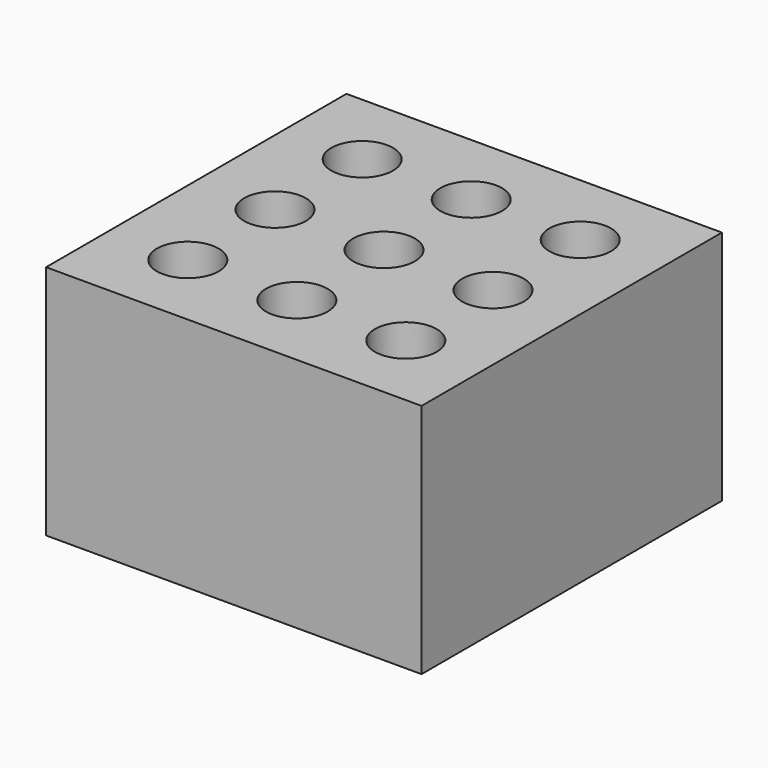
from build123d import *

# Parameters (mm, degrees)
F0_W      = 62
F0_H      = 62
F1_DEPTH  = 39
F4_DEPTH  = 8
F4_TAPER  = 22
F6_DEPTH  = 6
F6_TAPER  = 18
F9_DEPTH  = 6
F11_R     = 5.1
F12_DEPTH = 19


with BuildPart() as f1:
    # F0 (on Top) → F1 (new body)
    with BuildSketch(Plane.XY):
        Rectangle(F0_W, F0_H)
    extrude(amount=F1_DEPTH)

    # F3 (on Top) → F4 (cut)
    with BuildSketch(Plane.XY):
        with BuildLine():
            ThreePointArc((30.5, 29), (30.06066, 30.06066), (29, 30.5))
            Line((29, 30.5), (-29, 30.5))
            ThreePointArc((-29, 30.5), (-30.06066, 30.06066), (-30.5, 29))
            Line((-30.5, 29), (-30.5, -29))
            ThreePointArc((-30.5, -29), (-30.06066, -30.06066), (-29, -30.5))
            Line((-29, -30.5), (29, -30.5))
            ThreePointArc((29, -30.5), (30.06066, -30.06066), (30.5, -29))
            Line((30.5, -29), (30.5, 29))
        make_face()
    extrude(amount=F4_DEPTH, taper=F4_TAPER, mode=Mode.SUBTRACT)

    # F5 (on offset) → F6 (cut)
    with BuildSketch(Plane.XY.offset(8)):
        with BuildLine():
            Line((-9.5, -24.5), (-9.5, -11.5))
            ThreePointArc((-9.5, -11.5), (-10.085786, -10.085786), (-11.5, -9.5))
            Line((-11.5, -9.5), (-24.5, -9.5))
            ThreePointArc((-24.5, -9.5), (-25.914214, -10.085786), (-26.5, -11.5))
            Line((-26.5, -11.5), (-26.5, -24.5))
            ThreePointArc((-26.5, -24.5), (-25.914214, -25.914214), (-24.5, -26.5))
            Line((-24.5, -26.5), (-11.5, -26.5))
            ThreePointArc((-11.5, -26.5), (-10.085786, -25.914214), (-9.5, -24.5))
        make_face()
        with BuildLine():
            Line((8.5, -24.5), (8.5, -11.5))
            ThreePointArc((8.5, -11.5), (7.914214, -10.085786), (6.5, -9.5))
            Line((6.5, -9.5), (-6.5, -9.5))
            ThreePointArc((-6.5, -9.5), (-7.914214, -10.085786), (-8.5, -11.5))
            Line((-8.5, -11.5), (-8.5, -24.5))
            ThreePointArc((-8.5, -24.5), (-7.914214, -25.914214), (-6.5, -26.5))
            Line((-6.5, -26.5), (6.5, -26.5))
            ThreePointArc((6.5, -26.5), (7.914214, -25.914214), (8.5, -24.5))
        make_face()
        with BuildLine():
            Line((24.5, -9.5), (11.5, -9.5))
            ThreePointArc((11.5, -9.5), (10.085786, -10.085786), (9.5, -11.5))
            Line((9.5, -11.5), (9.5, -24.5))
            ThreePointArc((9.5, -24.5), (10.085786, -25.914214), (11.5, -26.5))
            Line((11.5, -26.5), (24.5, -26.5))
            ThreePointArc((24.5, -26.5), (25.914214, -25.914214), (26.5, -24.5))
            Line((26.5, -24.5), (26.5, -11.5))
            ThreePointArc((26.5, -11.5), (25.914214, -10.085786), (24.5, -9.5))
        make_face()
        with BuildLine():
            Line((26.5, -6.5), (26.5, 6.5))
            ThreePointArc((26.5, 6.5), (25.914214, 7.914214), (24.5, 8.5))
            Line((24.5, 8.5), (11.5, 8.5))
            ThreePointArc((11.5, 8.5), (10.085786, 7.914214), (9.5, 6.5))
            Line((9.5, 6.5), (9.5, -6.5))
            ThreePointArc((9.5, -6.5), (10.085786, -7.914214), (11.5, -8.5))
            Line((11.5, -8.5), (24.5, -8.5))
            ThreePointArc((24.5, -8.5), (25.914214, -7.914214), (26.5, -6.5))
        make_face()
        with BuildLine():
            Line((8.5, -6.5), (8.5, 6.5))
            ThreePointArc((8.5, 6.5), (7.914214, 7.914214), (6.5, 8.5))
            Line((6.5, 8.5), (-6.5, 8.5))
            ThreePointArc((-6.5, 8.5), (-7.914214, 7.914214), (-8.5, 6.5))
            Line((-8.5, 6.5), (-8.5, -6.5))
            ThreePointArc((-8.5, -6.5), (-7.914214, -7.914214), (-6.5, -8.5))
            Line((-6.5, -8.5), (6.5, -8.5))
            ThreePointArc((6.5, -8.5), (7.914214, -7.914214), (8.5, -6.5))
        make_face()
        with BuildLine():
            Line((-9.5, -6.5), (-9.5, 6.5))
            ThreePointArc((-9.5, 6.5), (-10.085786, 7.914214), (-11.5, 8.5))
            Line((-11.5, 8.5), (-24.5, 8.5))
            ThreePointArc((-24.5, 8.5), (-25.914214, 7.914214), (-26.5, 6.5))
            Line((-26.5, 6.5), (-26.5, -6.5))
            ThreePointArc((-26.5, -6.5), (-25.914214, -7.914214), (-24.5, -8.5))
            Line((-24.5, -8.5), (-11.5, -8.5))
            ThreePointArc((-11.5, -8.5), (-10.085786, -7.914214), (-9.5, -6.5))
        make_face()
        with BuildLine():
            Line((-9.5, 11.5), (-9.5, 24.5))
            ThreePointArc((-9.5, 24.5), (-10.085786, 25.914214), (-11.5, 26.5))
            Line((-11.5, 26.5), (-24.5, 26.5))
            ThreePointArc((-24.5, 26.5), (-25.914214, 25.914214), (-26.5, 24.5))
            Line((-26.5, 24.5), (-26.5, 11.5))
            ThreePointArc((-26.5, 11.5), (-25.914214, 10.085786), (-24.5, 9.5))
            Line((-24.5, 9.5), (-11.5, 9.5))
            ThreePointArc((-11.5, 9.5), (-10.085786, 10.085786), (-9.5, 11.5))
        make_face()
        with BuildLine():
            Line((8.5, 11.5), (8.5, 24.5))
            ThreePointArc((8.5, 24.5), (7.914214, 25.914214), (6.5, 26.5))
            Line((6.5, 26.5), (-6.5, 26.5))
            ThreePointArc((-6.5, 26.5), (-7.914214, 25.914214), (-8.5, 24.5))
            Line((-8.5, 24.5), (-8.5, 11.5))
            ThreePointArc((-8.5, 11.5), (-7.914214, 10.085786), (-6.5, 9.5))
            Line((-6.5, 9.5), (6.5, 9.5))
            ThreePointArc((6.5, 9.5), (7.914214, 10.085786), (8.5, 11.5))
        make_face()
        with BuildLine():
            Line((26.5, 11.5), (26.5, 24.5))
            ThreePointArc((26.5, 24.5), (25.914214, 25.914214), (24.5, 26.5))
            Line((24.5, 26.5), (11.5, 26.5))
            ThreePointArc((11.5, 26.5), (10.085786, 25.914214), (9.5, 24.5))
            Line((9.5, 24.5), (9.5, 11.5))
            ThreePointArc((9.5, 11.5), (10.085786, 10.085786), (11.5, 9.5))
            Line((11.5, 9.5), (24.5, 9.5))
            ThreePointArc((24.5, 9.5), (25.914214, 10.085786), (26.5, 11.5))
        make_face()
    extrude(amount=F6_DEPTH, taper=F6_TAPER, mode=Mode.SUBTRACT)

    # F8 (on offset) → F9 (cut)
    with BuildSketch(Plane.XY.offset(14)):
        with BuildLine():
            ThreePointArc((11.55, -23.45), (11.842893, -24.157107), (12.55, -24.45))
            Line((12.55, -24.45), (23.45, -24.45))
            ThreePointArc((23.45, -24.45), (24.157107, -24.157107), (24.45, -23.45))
            Line((24.45, -23.45), (24.45, -12.55))
            ThreePointArc((24.45, -12.55), (24.157107, -11.842893), (23.45, -11.55))
            Line((23.45, -11.55), (12.55, -11.55))
            ThreePointArc((12.55, -11.55), (11.842893, -11.842893), (11.55, -12.55))
            Line((11.55, -12.55), (11.55, -23.45))
        make_face()
        with BuildLine():
            Line((11.55, 5.45), (11.55, -5.45))
            ThreePointArc((11.55, -5.45), (11.842893, -6.157107), (12.55, -6.45))
            Line((12.55, -6.45), (23.45, -6.45))
            ThreePointArc((23.45, -6.45), (24.157107, -6.157107), (24.45, -5.45))
            Line((24.45, -5.45), (24.45, 5.45))
            ThreePointArc((24.45, 5.45), (24.157107, 6.157107), (23.45, 6.45))
            Line((23.45, 6.45), (12.55, 6.45))
            ThreePointArc((12.55, 6.45), (11.842893, 6.157107), (11.55, 5.45))
        make_face()
        with BuildLine():
            Line((11.55, 23.45), (11.55, 12.55))
            ThreePointArc((11.55, 12.55), (11.842893, 11.842893), (12.55, 11.55))
            Line((12.55, 11.55), (23.45, 11.55))
            ThreePointArc((23.45, 11.55), (24.157107, 11.842893), (24.45, 12.55))
            Line((24.45, 12.55), (24.45, 23.45))
            ThreePointArc((24.45, 23.45), (24.157107, 24.157107), (23.45, 24.45))
            Line((23.45, 24.45), (12.55, 24.45))
            ThreePointArc((12.55, 24.45), (11.842893, 24.157107), (11.55, 23.45))
        make_face()
        with BuildLine():
            Line((-6.45, -12.55), (-6.45, -23.45))
            ThreePointArc((-6.45, -23.45), (-6.157107, -24.157107), (-5.45, -24.45))
            Line((-5.45, -24.45), (5.45, -24.45))
            ThreePointArc((5.45, -24.45), (6.157107, -24.157107), (6.45, -23.45))
            Line((6.45, -23.45), (6.45, -12.55))
            ThreePointArc((6.45, -12.55), (6.157107, -11.842893), (5.45, -11.55))
            Line((5.45, -11.55), (-5.45, -11.55))
            ThreePointArc((-5.45, -11.55), (-6.157107, -11.842893), (-6.45, -12.55))
        make_face()
        with BuildLine():
            Line((-6.45, 5.45), (-6.45, -5.45))
            ThreePointArc((-6.45, -5.45), (-6.157107, -6.157107), (-5.45, -6.45))
            Line((-5.45, -6.45), (5.45, -6.45))
            ThreePointArc((5.45, -6.45), (6.157107, -6.157107), (6.45, -5.45))
            Line((6.45, -5.45), (6.45, 5.45))
            ThreePointArc((6.45, 5.45), (6.157107, 6.157107), (5.45, 6.45))
            Line((5.45, 6.45), (-5.45, 6.45))
            ThreePointArc((-5.45, 6.45), (-6.157107, 6.157107), (-6.45, 5.45))
        make_face()
        with BuildLine():
            Line((-6.45, 23.45), (-6.45, 12.55))
            ThreePointArc((-6.45, 12.55), (-6.157107, 11.842893), (-5.45, 11.55))
            Line((-5.45, 11.55), (5.45, 11.55))
            ThreePointArc((5.45, 11.55), (6.157107, 11.842893), (6.45, 12.55))
            Line((6.45, 12.55), (6.45, 23.45))
            ThreePointArc((6.45, 23.45), (6.157107, 24.157107), (5.45, 24.45))
            Line((5.45, 24.45), (-5.45, 24.45))
            ThreePointArc((-5.45, 24.45), (-6.157107, 24.157107), (-6.45, 23.45))
        make_face()
        with BuildLine():
            Line((-24.45, -12.55), (-24.45, -23.45))
            ThreePointArc((-24.45, -23.45), (-24.157107, -24.157107), (-23.45, -24.45))
            Line((-23.45, -24.45), (-12.55, -24.45))
            ThreePointArc((-12.55, -24.45), (-11.842893, -24.157107), (-11.55, -23.45))
            Line((-11.55, -23.45), (-11.55, -12.55))
            ThreePointArc((-11.55, -12.55), (-11.842893, -11.842893), (-12.55, -11.55))
            Line((-12.55, -11.55), (-23.45, -11.55))
            ThreePointArc((-23.45, -11.55), (-24.157107, -11.842893), (-24.45, -12.55))
        make_face()
        with BuildLine():
            Line((-24.45, 5.45), (-24.45, -5.45))
            ThreePointArc((-24.45, -5.45), (-24.157107, -6.157107), (-23.45, -6.45))
            Line((-23.45, -6.45), (-12.55, -6.45))
            ThreePointArc((-12.55, -6.45), (-11.842893, -6.157107), (-11.55, -5.45))
            Line((-11.55, -5.45), (-11.55, 5.45))
            ThreePointArc((-11.55, 5.45), (-11.842893, 6.157107), (-12.55, 6.45))
            Line((-12.55, 6.45), (-23.45, 6.45))
            ThreePointArc((-23.45, 6.45), (-24.157107, 6.157107), (-24.45, 5.45))
        make_face()
        with BuildLine():
            Line((-24.45, 23.45), (-24.45, 12.55))
            ThreePointArc((-24.45, 12.55), (-24.157107, 11.842893), (-23.45, 11.55))
            Line((-23.45, 11.55), (-12.55, 11.55))
            ThreePointArc((-12.55, 11.55), (-11.842893, 11.842893), (-11.55, 12.55))
            Line((-11.55, 12.55), (-11.55, 23.45))
            ThreePointArc((-11.55, 23.45), (-11.842893, 24.157107), (-12.55, 24.45))
            Line((-12.55, 24.45), (-23.45, 24.45))
            ThreePointArc((-23.45, 24.45), (-24.157107, 24.157107), (-24.45, 23.45))
        make_face()
    extrude(amount=F9_DEPTH, mode=Mode.SUBTRACT)

    # F11 (on offset) → F12 (cut)
    with BuildSketch(Plane.XY.offset(39)):
        with Locations((18, 18)):
            Circle(F11_R)
        with Locations((0, 18)):
            Circle(F11_R)
        with Locations((-18, 18)):
            Circle(F11_R)
        with Locations((-18, 0)):
            Circle(F11_R)
        Circle(F11_R)
        with Locations((18, 0)):
            Circle(F11_R)
        with Locations((18, -18)):
            Circle(F11_R)
        with Locations((0, -18)):
            Circle(F11_R)
        with Locations((-18, -18)):
            Circle(F11_R)
    extrude(amount=-F12_DEPTH, mode=Mode.SUBTRACT)


solid = f1.part
